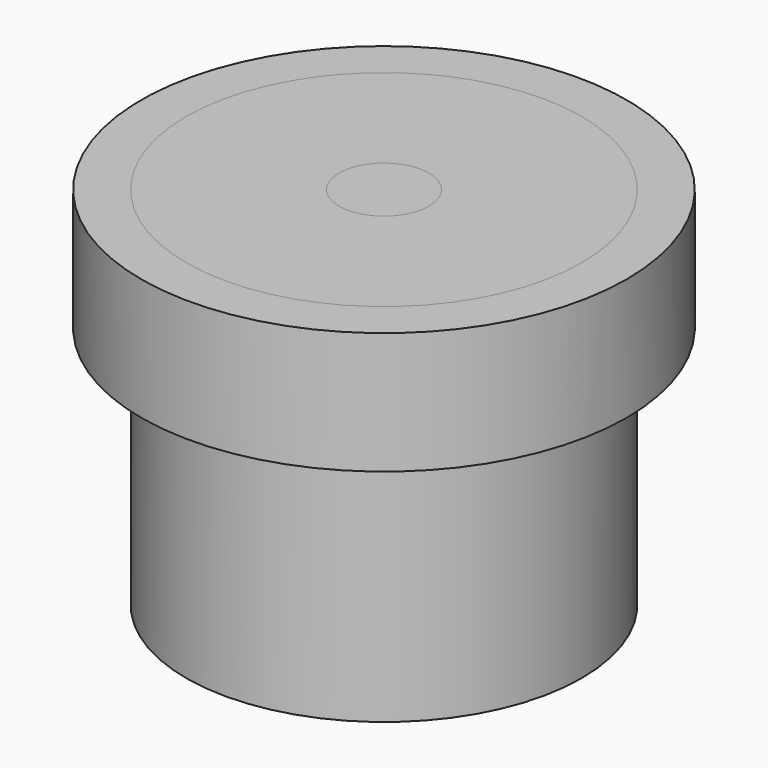
from build123d import *

# Parameters (mm, degrees)
F0_R     = 25.287927835
F0_R_2   = 25.2654785995
F2_DEPTH = 12.7
F1_R     = 20.6121053544
F1_R_2   = 4.679734569
F3_DEPTH = 38.1


# Not quite as in the source:
# - a feature of the source that left no trace in its solid (it failed there, or was rolled back) is left out
# - a feature names something its author has since deleted; it is built from what else it names


with BuildPart() as f2:
    # F0 (on Top) → F2 (new body)
    with BuildSketch(Plane.XY):
        Circle(F0_R)
        Circle(F0_R_2, mode=Mode.SUBTRACT)
        Circle(F0_R_2)
    extrude(amount=F2_DEPTH)


with BuildPart() as f2b:
    # F1 (on Top) → F2, piece 2 (new body)
    with BuildSketch(Plane.XY):
        Circle(F1_R)
        Circle(F1_R_2, mode=Mode.SUBTRACT)
    extrude(amount=F2_DEPTH)


with BuildPart() as f3:
    # F3 (new): a face of the model
    f3_faces = [f2b.part.faces().sort_by_distance(p)[0] for p in [
        (-20.0291069756, 0, 12.7),
    ]]
    extrude(f3_faces, amount=-F3_DEPTH)


solid = Compound([f2.part, f2b.part, f3.part])
